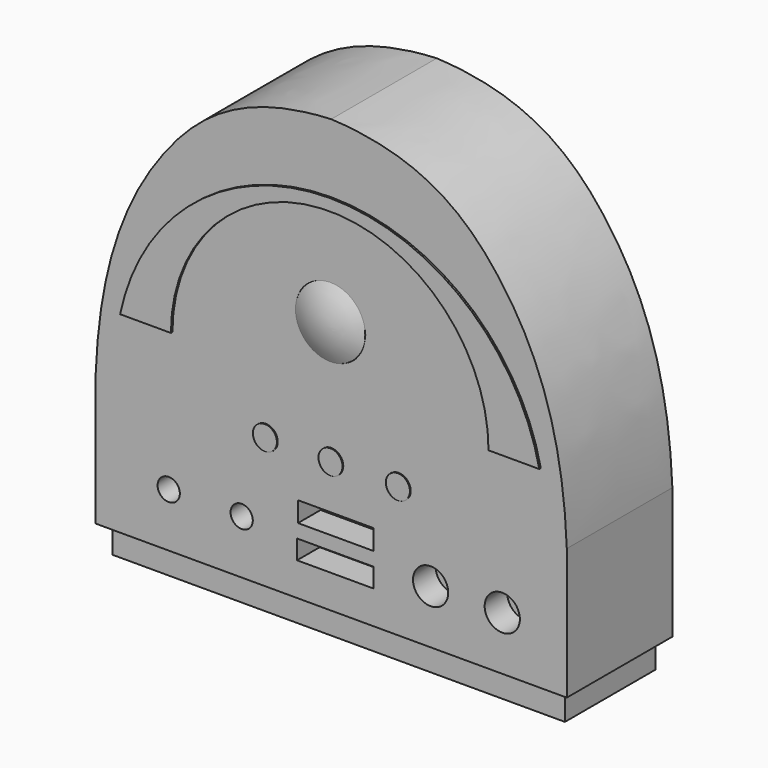
from build123d import *

# Parameters (mm, degrees)
F1_DEPTH     = 35.56
F2_W         = 20.4069074243
F2_H         = 5.429463461
F2_W_2       = 20.6557726488
F2_H_2       = 5.1806047559
F2_R         = 4.7472786305
F2_R_2       = 2.9967281819
F3_DEPTH     = 7.62
F5_DEPTH     = 0.254
F4_R         = 3.2448006106
F6_DEPTH     = 0.254
F7_T         = 2.54
F7_T3_DEPTH  = 12.7
F7_T5_DEPTH  = 25.7357726488
F7_T7_DEPTH  = 10.2606047559
F7_T9_DEPTH  = 25.4869074243
F7_T11_DEPTH = 10.509463461
F9_W         = 121.92
F9_H         = 30.48
F10_DEPTH    = 12.7


# Not quite as in the source:
# - a shell that OpenCascade refuses in one call is made with other operations: the cavity is built on its own and cut out


with BuildPart() as f1:
    # F0 (on Front) → F1 (new body)
    with BuildSketch(Plane.XZ):
        with BuildLine():
            Line((-63.5, -52.164846403), (0, -52.164846403))
            Line((0, -52.164846403), (63.5, -52.164846403))
            Line((63.5, -52.164846403), (63.5, -16.7983658612))
            add(Edge.make_bspline(
                [(63.5, -16.7983658612), (62.4360478279, 10.32030946), (49.129273617, 44.0268624364), (23.4670229256, 63.3222609758), (0, 64.4457638264)],
                knots=[0, 0, 0, 0, 0.5242691479, 1, 1, 1, 1], degree=3))
            add(Edge.make_bspline(
                [(-63.5, -16.7983658612), (-62.4360478279, 10.32030946), (-49.129273617, 44.0268624364), (-23.4670229256, 63.3222609758), (0, 64.4457638264)],
                knots=[0, 0, 0, 0, 0.5242691479, 1, 1, 1, 1], degree=3))
            Line((-63.5, -16.7983658612), (-63.5, -52.164846403))
        make_face()
    extrude(amount=F1_DEPTH)

    # F2 (on face) → F3 (cut)
    with BuildSketch(Plane.XZ.offset(35.56)):
        with Locations((1.2443242595, -31.5884416923)):
            Rectangle(F2_W, F2_H)
        with Locations((1.1198916472, -40.6264439225)):
            Rectangle(F2_W_2, F2_H_2)
        with Locations((26.7892014235, -37.6602374017)):
            Circle(F2_R)
        with Locations((46.0982057871, -37.6602374017)):
            Circle(F2_R)
        with Locations((-24.1335762036, -37.6602374017)):
            Circle(F2_R_2)
        with Locations((-43.8001863658, -37.6602374017)):
            Circle(F2_R_2)
    extrude(amount=-F3_DEPTH, mode=Mode.SUBTRACT)

    # F7: shell of thickness 2.54, made by hand


with BuildPart() as f5:
    # F4 (on face) → F5 (new body)
    with BuildSketch(Plane.XZ.offset(35.56)):
        with BuildLine():
            Line((-56.4922876656, 0), (-42.8047291934, 0))
            ThreePointArc((-42.8047291934, 0), (0, 42.8047291934), (42.8047291934, 0))
            Line((42.8047291934, 0), (56.4922876656, 0))
            ThreePointArc((56.4922876656, 0), (0, 45.95054916), (-56.4922876656, 0))
        make_face()
    extrude(amount=F5_DEPTH)


with BuildPart() as f5b:
    # F4 (on face) → F5, piece 2 (new body)
    with BuildSketch(Plane.XZ.offset(35.56)):
        with Locations((-17.6693946123, -16.7983658612)):
            Circle(F4_R)
    extrude(amount=F5_DEPTH)


with BuildPart() as f5c:
    # F4 (on face) → F5, piece 3 (new body)
    with BuildSketch(Plane.XZ.offset(35.56)):
        with Locations((0, -16.7983658612)):
            Circle(F4_R)
    extrude(amount=F5_DEPTH)


with BuildPart() as f5d:
    # F4 (on face) → F5, piece 4 (new body)
    with BuildSketch(Plane.XZ.offset(35.56)):
        with Locations((18.1671231985, -16.7983658612)):
            Circle(F4_R)
    extrude(amount=F5_DEPTH)


with BuildPart() as f6:
    # F6 (new): a face of the model
    f6_faces = [f5.part.faces().sort_by_distance(p)[0] for p in [
        (-49.6485084295, -35.814, 1.2197117377),
    ]]
    extrude(f6_faces, amount=F6_DEPTH)


with BuildPart() as f7_core1:
    # F7_t2: copy of F1
    add(f1.part)

    # the walls: a layer under each face that stays
    f7_faces = [f7_core1.faces().sort_by_distance(p)[0] for p in [
        (-63.5, -17.78, -34.4816061321),
        (0, -35.56, 6.1404587117),
        (63.5, -17.78, -34.4816061321),
        (0, 0, 6.1404587117),
        (-46.5057501218, -17.78, 39.7718854475),
        (46.5057501218, -17.78, 39.7718854475),
        (1.1198916472, -31.75, -38.0361415446),
        (-9.2079946771, -31.75, -40.6264439225),
        (1.1198916472, -31.75, -43.2167463005),
        (11.4477779716, -31.75, -40.6264439225),
        (-46.7969145477, -31.75, -37.6602374017),
        (-27.1303043855, -31.75, -37.6602374017),
        (22.041922793, -31.75, -37.6602374017),
        (41.3509271565, -31.75, -37.6602374017),
        (1.2443242595, -31.75, -28.8737099618),
        (-8.9591294527, -31.75, -31.5884416923),
        (1.2443242595, -31.75, -34.3031734228),
        (11.4477779716, -31.75, -31.5884416923),
        (1.1198916472, -27.94, -40.6264439225),
        (-43.8001863658, -27.94, -37.6602374017),
        (-24.1335762036, -27.94, -37.6602374017),
        (26.7892014235, -27.94, -37.6602374017),
        (46.0982057871, -27.94, -37.6602374017),
        (1.2443242595, -27.94, -31.5884416923),
    ]]
    thicken(f7_faces, amount=-F7_T, mode=Mode.SUBTRACT)

    # F7_s4 → F7_t3 (cut)
    with BuildSketch(Plane.XZ.offset(25.4)):
        Polygon((11.4223779716, -38.0615415446), (11.4477779716, -35.4961415446), (13.9877779716, -35.4961415446), (13.9877779716, -38.0361415446), align=None)
        Polygon((-9.1825946771, -38.0615415446), (-9.2079946771, -35.4961415446), (-11.7479946771, -35.4961415446), (-11.7479946771, -38.0361415446), align=None)
        Polygon((-9.1825946771, -43.1913463005), (-11.7479946771, -43.2167463005), (-11.7479946771, -45.7567463005), (-9.2079946771, -45.7567463005), align=None)
        Polygon((11.4223779716, -43.1913463005), (11.4477779716, -45.7567463005), (13.9877779716, -45.7567463005), (13.9877779716, -43.2167463005), align=None)
        Polygon((11.4223779716, -28.8991099618), (11.4477779716, -26.3337099618), (13.9877779716, -26.3337099618), (13.9877779716, -28.8737099618), align=None)
        Polygon((-8.9337294527, -28.8991099618), (-8.9591294527, -26.3337099618), (-11.4991294527, -26.3337099618), (-11.4991294527, -28.8737099618), align=None)
        Polygon((-8.9337294527, -34.2777734228), (-11.4991294527, -34.3031734228), (-11.4991294527, -36.8431734228), (-8.9591294527, -36.8431734228), align=None)
        Polygon((11.4223779716, -34.2777734228), (11.4477779716, -36.8431734228), (13.9877779716, -36.8431734228), (13.9877779716, -34.3031734228), align=None)
    extrude(amount=F7_T3_DEPTH, mode=Mode.SUBTRACT)

    # F7_s6 → F7_t5 (cut)
    with BuildSketch(Plane.YZ.offset(-11.7479946771)):
        Polygon((-27.9654, -38.0615415446), (-27.94, -35.4961415446), (-25.4, -35.4961415446), (-25.4, -38.0361415446), align=None)
        Polygon((-27.9654, -43.1913463005), (-27.94, -45.7567463005), (-25.4, -45.7567463005), (-25.4, -43.2167463005), align=None)
    extrude(amount=F7_T5_DEPTH, mode=Mode.SUBTRACT)

    # F7_s8 → F7_t7 (cut)
    with BuildSketch(Plane.XY.offset(-45.7567463005)):
        Polygon((-9.1825946771, -27.9654), (-11.7479946771, -27.94), (-11.7479946771, -25.4), (-9.2079946771, -25.4), align=None)
        Polygon((11.4223779716, -27.9654), (13.9877779716, -27.94), (13.9877779716, -25.4), (11.4477779716, -25.4), align=None)
    extrude(amount=F7_T7_DEPTH, mode=Mode.SUBTRACT)

    # F7_s10 → F7_t9 (cut)
    with BuildSketch(Plane.YZ.offset(-11.4991294527)):
        Polygon((-27.9654, -28.8991099618), (-27.94, -26.3337099618), (-25.4, -26.3337099618), (-25.4, -28.8737099618), align=None)
        Polygon((-27.9654, -34.2777734228), (-27.94, -36.8431734228), (-25.4, -36.8431734228), (-25.4, -34.3031734228), align=None)
    extrude(amount=F7_T9_DEPTH, mode=Mode.SUBTRACT)

    # F7_s12 → F7_t11 (cut)
    with BuildSketch(Plane.XY.offset(-36.8431734228)):
        Polygon((-8.9337294527, -27.9654), (-11.4991294527, -27.94), (-11.4991294527, -25.4), (-8.9591294527, -25.4), align=None)
        Polygon((11.4223779716, -27.9654), (13.9877779716, -27.94), (13.9877779716, -25.4), (11.4477779716, -25.4), align=None)
    extrude(amount=F7_T11_DEPTH, mode=Mode.SUBTRACT)

    # F7_s13 → F7_t14 (revolve, cut)
    with BuildSketch(Plane.XY.offset(-37.6602374017)):
        Polygon((-40.8288581839, -27.9654), (-38.2634581839, -27.94), (-38.2634581839, -25.4), (-40.8034581839, -25.4), align=None)
    revolve(axis=Axis((-43.8001863658, -27.94, -37.6602374017), (0, -1, 0)), mode=Mode.SUBTRACT)

    # F7_s15 → F7_t16 (revolve, cut)
    with BuildSketch(Plane.XY.offset(-37.6602374017)):
        Polygon((-21.1622480217, -27.9654), (-18.5968480217, -27.94), (-18.5968480217, -25.4), (-21.1368480217, -25.4), align=None)
    revolve(axis=Axis((-24.1335762036, -27.94, -37.6602374017), (0, -1, 0)), mode=Mode.SUBTRACT)

    # F7_s17 → F7_t18 (revolve, cut)
    with BuildSketch(Plane.XY.offset(-37.6602374017)):
        Polygon((31.5110800541, -27.9654), (34.0764800541, -27.94), (34.0764800541, -25.4), (31.5364800541, -25.4), align=None)
    revolve(axis=Axis((26.7892014235, -27.94, -37.6602374017), (0, -1, 0)), mode=Mode.SUBTRACT)

    # F7_s19 → F7_t20 (revolve, cut)
    with BuildSketch(Plane.XY.offset(-37.6602374017)):
        Polygon((50.8200844176, -27.9654), (53.3854844176, -27.94), (53.3854844176, -25.4), (50.8454844176, -25.4), align=None)
    revolve(axis=Axis((46.0982057871, -27.94, -37.6602374017), (0, -1, 0)), mode=Mode.SUBTRACT)


with BuildPart() as f1_1:
    add(f1.part)

    # what is left inside the walls is the cavity
    f7_cavity = [f7_core1.part.solids().sort_by_distance(p)[0] for p in [
        (0, -2.5654, -14.142306),
    ]]
    add(f7_cavity, mode=Mode.SUBTRACT)


with BuildPart() as f10:
    # F9 (on offset) → F10 (new body)
    with BuildSketch(Plane(origin=(0, 0, -47.084846403), x_dir=(1, 0, 0), z_dir=(0, 0, -1))):
        with Locations((0, 17.78)):
            Rectangle(F9_W, F9_H)
    extrude(amount=F10_DEPTH)


with BuildPart() as f13:
    # F12 (on offset) → F13 (revolve)
    with BuildSketch(Plane(origin=(0, 0, 16.415153597), x_dir=(1, 0, 0), z_dir=(0, 0, -1))):
        with BuildLine():
            ThreePointArc((9.4112261052, 35.8505937442), (4.8575423267, 37.6490778959), (0, 38.2613390684))
            Line((0, 38.2613390684), (0, 37.6547761261))
            ThreePointArc((0, 37.6547761261), (4.1366254111, 37.1982365786), (8.074131848, 35.8505937442))
            Line((8.074131848, 35.8505937442), (9.4112261052, 35.8505937442))
        make_face()
    revolve(axis=Axis((0, -35.8350872993, 16.415153597), (0, 1, 0)))


solid = Compound([f5.part, f5b.part, f5c.part, f5d.part, f6.part, f1_1.part, f10.part, f13.part])
